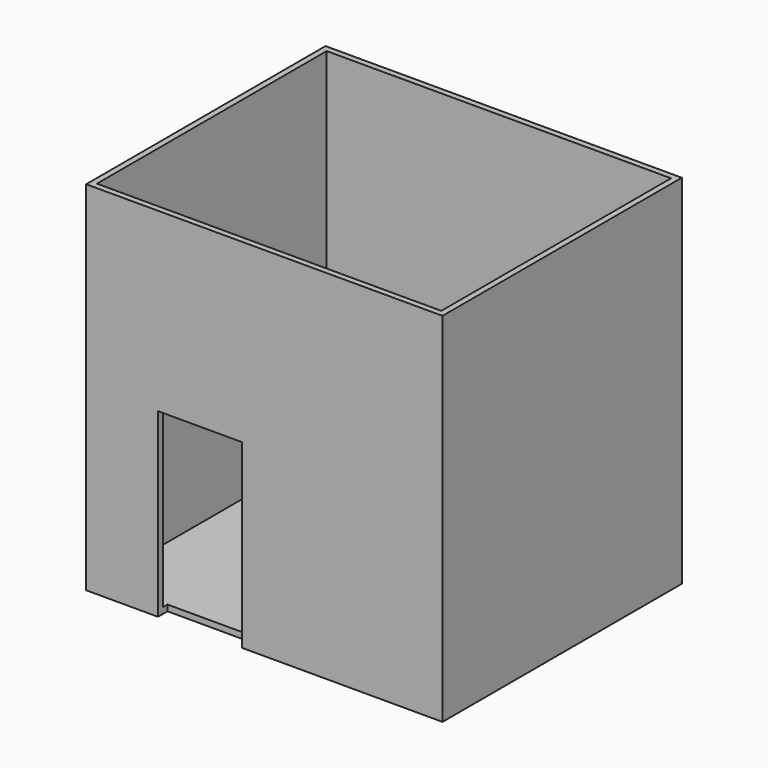
from build123d import *

# Parameters (mm, degrees)
F0_W      = 152.267947793
F0_H      = 151.1743441224
F1_DEPTH  = 101.6
F2_SIZE   = 50.8
F3_SIZE   = 50.79999
F4_SIZE   = 50.8
F5_T      = -2.54
F7_W      = 151.2815654278
F7_H      = 151.7730951309
F8_DEPTH  = 127
F9_T      = -2.54
F10_W     = 35.6509871781
F10_H     = 76.8820419908
F11_DEPTH = 0.0254
F12_DEPTH = 2.54
F13_DEPTH = 2.54


# Not quite as in the source:
# - a fillet or chamfer is up to 0.001 mm smaller than in the source, because OpenCascade refuses the exact size


with BuildPart() as f1:
    # F0 (on Top) → F1 (new body)
    with BuildSketch(Plane.XY):
        with Locations((-0.6233751774, 0.4115886986)):
            Rectangle(F0_W, F0_H)
    extrude(amount=F1_DEPTH)

    # F2
    f2_edges = [f1.edges().sort_by_distance(p)[0] for p in [
        (-76.757349, 0.411589, 101.6),
        (-0.623375, -75.175583, 101.6),
        (75.510599, 0.411589, 101.6),
        (-0.623375, 75.998761, 101.6),
    ]]
    chamfer(f2_edges, length=F2_SIZE)

    # F3 (size 50.8 in the source; OpenCascade refuses exactly that, so slightly less here)
    f3_edges = [f1.edges().sort_by_distance(p)[0] for p in [
        (-0.623375, -75.175583, 0),
    ]]
    chamfer(f3_edges, length=F3_SIZE)

    # F4
    f4_edges = [f1.edges().sort_by_distance(p)[0] for p in [
        (75.510599, 75.998761, 25.4),
    ]]
    chamfer(f4_edges, length=F4_SIZE)

    # F5
    f5_openings = [f1.faces().sort_by_distance(p)[0] for p in [
        (-0.623375, 0.411589, 101.6),
    ]]
    offset(amount=F5_T, openings=f5_openings)


with BuildPart() as f8:
    # F7 (on Front) → F8 (new body)
    with BuildSketch(Plane.XZ):
        with Locations((-0.3735423088, -0.9954944253)):
            Rectangle(F7_W, F7_H)
    extrude(amount=F8_DEPTH)

    # F9
    f9_openings = [f8.faces().sort_by_distance(p)[0] for p in [
        (-0.373542, -63.5, 74.891053),
    ]]
    offset(amount=F9_T, openings=f9_openings)

    # F10 (on face) → F11 (join)
    with BuildSketch(Plane.XZ.offset(127)):
        with Locations((-27.7109388262, -38.4410209954)):
            Rectangle(F10_W, F10_H)
    extrude(amount=F11_DEPTH)

    # F12 (cut): a face of the model
    f12_faces = [f8.faces().sort_by_distance(p)[0] for p in [
        (-27.7109388262, -127.0254, -38.4410209954),
    ]]
    extrude(f12_faces, amount=-F12_DEPTH, mode=Mode.SUBTRACT)

    # F13 (cut): a face of the model
    f13_faces = [f8.faces().sort_by_distance(p)[0] for p in [
        (-27.7109388262, -124.4854, -38.4410209954),
    ]]
    extrude(f13_faces, amount=-F13_DEPTH, mode=Mode.SUBTRACT)


solid = f8.part
